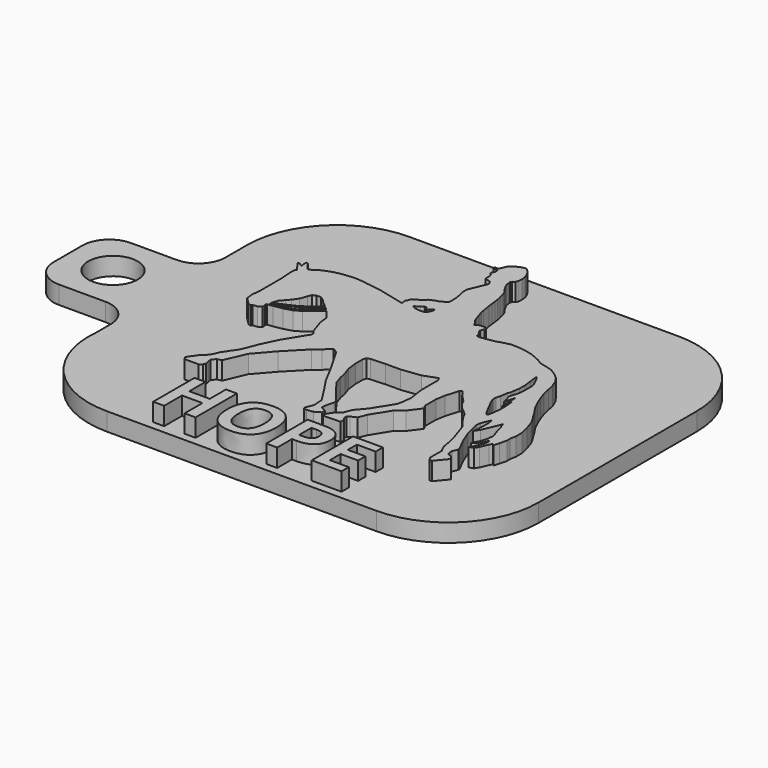
from build123d import *

# Parameters (mm, degrees)
F0_R         = 2.75
F1_DEPTH     = 2
F3_TEXT_SIZE = 8.0529393421
F4_DEPTH     = 2
F5_DEPTH     = 2


# Not quite as in the source:
# - Text() gives the source's letters only with a copy of the font that has no kerning and outlines rounded to 1/6400 em; it was checked with that copy


with BuildPart() as f1:
    # F0 (on Top) → F1 (new body)
    with BuildSketch(Plane.XY):
        with BuildLine():
            ThreePointArc((-13.1507226788, -10), (-10.6170467948, -17.7082039325), (-3.2008483077, -21))
            Line((-3.2008483077, -21), (26.7991516923, -21))
            ThreePointArc((26.7991516923, -21), (33.8702195042, -18.0710678119), (36.7991516923, -11))
            Line((36.7991516923, -11), (36.7991516923, 11))
            ThreePointArc((36.7991516923, 11), (33.8702195042, 18.0710678119), (26.7991516923, 21))
            Line((26.7991516923, 21), (-3.2008483077, 21))
            ThreePointArc((-3.2008483077, 21), (-10.2719161196, 18.0710678119), (-13.2008483077, 11))
            Line((-13.2008483077, 11), (-13.2008483077, 8))
            ThreePointArc((-13.2008483077, 8), (-14.0795279641, 5.8786796564), (-16.2008483077, 5))
            Line((-16.2008483077, 5), (-21.3089559265, 5))
            ThreePointArc((-21.3089559265, 5), (-23.43027627, 4.1213203436), (-24.3089559265, 2))
            Line((-24.3089559265, 2), (-24.3089559265, -2))
            ThreePointArc((-24.3089559265, -2), (-23.43027627, -4.1213203436), (-21.3089559265, -5))
            Line((-21.3089559265, -5), (-16.1507226788, -5))
            ThreePointArc((-16.1507226788, -5), (-14.0294023352, -5.8786796564), (-13.1507226788, -8))
            Line((-13.1507226788, -8), (-13.1507226788, -10))
        make_face()
        with Locations((-19.3089559265, 0)):
            Circle(F0_R, mode=Mode.SUBTRACT)
    extrude(amount=F1_DEPTH)

    # F3 (on face) → F4 (join)
    with BuildSketch(Plane.XY.offset(2)):
        with Locations((0.5135238171, -20.096231252)):
            Text('HOPE', F3_TEXT_SIZE, font='Open Sans', font_style=FontStyle.BOLD, text_align=(TextAlign.LEFT, TextAlign.BOTTOM))
    extrude(amount=F4_DEPTH)

    # F2 (on face) → F5 (join)
    with BuildSketch(Plane.XY.offset(2)):
        Polygon((14.4057357684, -12.9295000806), (16.3045506924, -12.8705985844), (16.2954782047, -12.3983173033), (16.0806663334, -12.0984232053), (16.0806663334, -11.8137812242), (16.300862655, -11.6041181609), (16.9360265136, -11.3009717315), (17.3037418711, -10.3799057515), (18.5667234945, -8.336847648), (19.4170251489, -7.6700611971), (20.3772753385, -6.3978997059), (20.1262235641, -5.9626172297), (20.1262235641, -4.43818653), (20.2957785632, -3.396378751), (20.734641701, -1.9284236478), (20.9365651874, -1.7577570332), (21.4741043746, -2.4432395585), (22.2038775682, -3.195283236), (22.4202004258, -3.6323247982), (22.9209531099, -4.2708963156), (23.7911492586, -4.9933143891), (24.1744478729, -5.7404879736), (25.1152147488, -6.9401758645), (25.5047673759, -8.102159261), (25.8359651324, -9.0900778816), (26.0207999805, -9.8925542569), (26.1829775535, -10.8235611911), (26.3887103647, -11.3350939359), (26.5676892823, -11.6454139352), (26.5676892823, -13.2674037658), (26.7900731415, -13.6529807933), (27.0690526813, -13.6529807933), (28.1546071398, -12.3415887356), (27.8195337628, -11.91429534), (27.6246890426, -11.9076147676), (27.4183303118, -11.7746600881), (27.3406576146, -11.6189256126), (27.289854211, -11.3983582705), (27.289854211, -11.1325758151), (27.5425345508, -10.546027472), (27.5135968314, -10.3799057515), (26.8309513895, -9.0288437401), (26.2567778986, -7.6012224477), (26.0578238236, -6.7374462358), (25.8793570101, -5.9626172297), (25.9441418617, -5.4701659828), (26.3887103647, -4.43818653), (26.4952767074, -5.1568056859), (26.4448728412, -6.6268783994), (26.3512693346, -7.0590674877), (26.7444010824, -6.4693694003), (27.5868289173, -4.4288262725), (27.7840252444, -4.9476545199), (28.0780084431, -5.9626172297), (28.3293427293, -6.6593339926), (28.2371323556, -7.4789840728), (28.001123842, -8.18628259), (27.6055055558, -8.91732222), (28.0312057585, -8.5834981874), (28.3802725508, -8.18628259), (28.5535737633, -7.6066066558), (28.6533644503, -7.610028144), (28.6533644503, -8.18628259), (28.1435307115, -9.3697626144), (27.918882668, -9.6224909648), (28.4013585813, -9.4954507706), (28.6819663905, -9.0415264633), (29.050398618, -8.18628259), (29.2314309627, -7.8517636284), (29.4054470205, -8.0243692113), (29.5858703554, -7.4208704612), (29.7829452902, -6.6268783994), (29.7763942349, -6.1731628859), (29.8888737889, -5.4701659828), (29.8888737889, -4.6576105355), (29.6704190609, -3.7091705624), (29.3347928673, -2.7080425061), (29.0434602648, -2.1314497571), (28.7286803838, -1.6768321487), (28.2960847475, -0.9267824817), (27.8613511473, -0.3198605264), (27.3939305483, 0.6458187127), (27.0699299872, 1.4514116338), (26.8065321311, 2.2446609869), (26.5914796644, 3.17832975), (26.4157085241, 3.9414552589), (26.0975691721, 4.7324749074), (25.7041398436, 5.2817328833), (25.1186332892, 5.7565801296), (24.4813356549, 6.150546018), (23.8515025278, 6.3388423371), (22.9791355302, 6.5553705336), (22.3837151171, 6.9234486801), (21.3705125394, 7.3599282554), (20.5815926346, 7.5557442418), (19.7165142745, 7.6941568404), (18.8413587665, 7.7241629896), (18.1382677906, 7.5622196381), (17.2448255293, 7.3034347474), (16.3118303177, 7.1409108247), (15.8028327753, 7.0781577004), (15.4516413608, 7.117666623), (15.3766200171, 7.376674167), (15.2874930965, 7.5982787718), (15.0793138891, 7.8889131546), (15.0296255656, 8.0652720289), (15.0862894952, 8.2935644314), (15.1866925525, 8.5351212571), (15.1628451422, 8.7285502439), (15.0607703254, 8.8532911029), (14.6830938756, 8.8532911029), (14.3462475389, 8.8090412319), (13.9642081238, 8.6108921573), (13.9168873429, 8.7285502439), (13.7182632894, 9.0058448879), (13.5212177411, 9.257121973), (13.3323129267, 9.7268136943), (13.1886444769, 10.2228220367), (12.9617797656, 10.8995291345), (12.9220215604, 11.222012341), (12.7522886811, 12.1963917492), (12.6947659129, 12.6629652935), (12.6373895197, 13.1283515742), (12.5825373734, 13.5732634076), (12.4628860503, 14.0927399082), (12.3358950912, 14.6440820693), (12.184023687, 15.0216941566), (11.8444845447, 15.4957172366), (11.5512409369, 16.004153411), (11.4555447903, 16.2420916973), (11.4297282051, 16.4514928789), (11.4029068374, 16.6690439634), (11.3867729017, 16.7999081028), (11.4582277826, 16.9657767335), (11.7187928736, 17.1701057165), (11.81913508, 17.4030306642), (11.8690588013, 17.846798328), (11.8006470133, 18.4016939184), (11.6284643142, 18.829807879), (11.3886492327, 19.2456077784), (11.0933948308, 19.5535104722), (10.8797093853, 19.6888073356), (10.5026904296, 19.6423255446), (10.0986134797, 19.4798102654), (9.6864081913, 19.2420683973), (9.4014372543, 19.0186009269), (9.0297050774, 18.1556968618), (8.6688981794, 18.1556968618), (8.575363435, 18.101750138), (8.5913146254, 17.9723682655), (8.8844563685, 17.925465566), (9.1159679477, 17.8994205868), (9.1672958909, 17.7717991173), (9.1672958909, 17.4858884987), (9.0056583988, 17.2244161367), (9.0056583988, 17.1079486746), (9.0216090903, 17.0386973768), (9.2548581452, 16.8271699), (9.2950100008, 16.501493752), (9.2950100008, 16.0436237693), (9.3934232773, 15.9181248609), (9.8117959588, 15.871058067), (9.9814711139, 15.7979633659), (10.1616944747, 15.3498571551), (9.9239231119, 14.7979171072), (9.334008789, 13.428545557), (9.334008789, 12.7822692709), (9.533021627, 11.9182379339), (9.5952630636, 11.4133907482), (9.5952630636, 11.1038507894), (9.5952630636, 10.5683606976), (8.8377370251, 10.1314530193), (8.4686949849, 10.0464513525), (7.862482393, 9.7754532312), (7.773434688, 9.5687462755), (7.1687237712, 9.2199756336), (6.6696759257, 8.9321468007), (6.5858433046, 8.5943948905), (6.4547806883, 8.3823818766), (6.5029077057, 7.992018307), (6.5264196133, 7.8899393401), (6.3388443612, 7.9110414964), (5.2770058221, 8.1745979864), (4.3924666627, 8.3941474071), (3.5704599901, 8.5981757837), (2.6782433787, 8.7409305045), (1.9472041167, 8.8231721893), (1.1549399933, 8.9499345049), (0.4360472958, 8.9999223128), (-0.3550298657, 8.9431121583), (-1.083578395, 8.8532911029), (-1.7623456147, 8.6969502562), (-2.4313051254, 8.4726829082), (-3.0800345292, 8.1745979864), (-3.5510911003, 7.837183732), (-3.8549916855, 7.735301664), (-4.5147598108, 8.5766533857), (-4.6581168893, 8.6652741428), (-4.7388332486, 8.5347035874), (-4.6581168893, 7.8800042569), (-5.1091981368, 8.1588545378), (-5.2491402967, 8.1745979864), (-5.2741511807, 8.0738320349), (-4.9507311765, 7.6613992925), (-4.4976170656, 7.0835775961), (-4.6094932536, 6.9026014455), (-4.6581168893, 6.4703901298), (-4.5513651165, 5.0638681278), (-4.5513651165, 3.0954778194), (-4.5513651165, 1.9436620058), (-4.6581168893, 0.9947546798), (-4.5619914308, 0.2150704386), (-3.7474798462, -0.5943234321), (-3.4712990843, -0.6253936801), (-3.3903366707, -0.4944250957), (-2.8851934087, -0.4321471566), (-2.5077828025, -0.2144733298), (-2.5077828025, -0.0057062971), (-2.5319425578, 0.0991853563), (-2.5757992459, 0.2300039925), (-2.5077828025, 0.3878909582), (-1.9108937122, 0.4614800273), (-0.8987553301, 0.6458187127), (0, 0.9061425298), (0.7114020668, 1.3164479313), (2.3607970983, 2.6098645129), (3.1293474968, 1.629791096), (3.2593631487, 0.5752197428), (3.7923315989, -1.0145538767), (4.0943801749, -1.3997332749), (4.0632066396, -1.6768321487), (2.5680158287, -4.0955226868), (1.6779805301, -5.9481193312), (0.9921386372, -7.6900362037), (0.5374790689, -8.336847648), (-0.0548549726, -9.2235639258), (-0.431542634, -10.097971186), (-1.0948275449, -10.7212318107), (-1.8477179687, -11.7997636751), (-1.6525899991, -12.1380834737), (-0.0900417419, -12.1380834737), (0.2038573346, -11.9076147676), (0.3361684251, -11.6004802633), (0.2267933478, -11.1256189671), (0.1865181403, -10.7989422977), (0.5374790689, -10.3799057515), (1.0402089683, -10.2641116828), (2.0574387163, -7.9028103501), (3.7640798837, -5.9423525818), (5.8369720424, -3.8145952286), (6.5262070857, -3.2741134055), (7.2511202059, -2.5279033566), (7.8156586153, -2.8768908061), (9.2243542895, -5.3193373606), (10.4674790055, -7.6557914726), (11.4393364638, -9.1057261452), (12.4628860503, -10.7212318107), (12.542760931, -11.8435025215), (12.1880317868, -12.704298012), (12.2453598306, -12.8752999008), (12.5538124515, -12.9654358891), (13.2664684206, -12.8775741905), (13.9168873429, -12.5024411827), (13.9168873429, -12.0695345104), (13.5212177411, -11.9076147676), (13.3323129267, -11.7698712274), (13.3323129267, -11.4510944113), (13.5909453758, -10.4090942619), (13.5491946712, -10.0704496726), (13.0443628877, -9.4802035019), (12.1477702633, -8.336847648), (11.3876733474, -7.2756931705), (11.0933948308, -6.3978997059), (10.8797093853, -5.4701659828), (10.6073017845, -4.6576105355), (10.4674790055, -3.5234924871), (10.4674790055, -2.5159725919), (10.5888666585, -2.1214617882), (10.9651694074, -2.0304208156), (12.5497952104, -1.9438075833), (14.2243178561, -1.9438075833), (16.3319073617, -1.6839677701), (17.8187675774, -1.1354173766), (18.035300076, -1.4241281897), (18.035300076, -2.4634872098), (18.035300076, -3.8781699259), (18.2807035744, -5.523821339), (18.1507840753, -6.6786645912), (18.035300076, -7.1839080192), (16.6555959731, -9.395503439), (15.7172307372, -10.4874065146), (15.3705142438, -11.3918855786), (14.8881245404, -11.7235276848), (14.4660342485, -12.3415887356), (14.2097650096, -12.756141834), align=None)
        Polygon((0.7803506547, 2.1377503983), (1.9207079895, 3.031991655), (2.1353650372, 2.8217774816), (0.7837259327, 1.6832037363), (-0.0899588704, 1.1401023949), (-1.0226764716, 0.8173899841), (-2.3492628576, 0.6119563146), (-2.3961719126, 0.671775837), (-1.1930471958, 1.0943717908), (0, 1.6577552306), align=None, mode=Mode.SUBTRACT)
        Polygon((1.1432619067, 3.6654123105), (1.7351189163, 3.2034749165), (0.6813245127, 2.3806493264), (-0.1848077227, 1.8176630838), (-1.2241665972, 1.32685469), (-2.3790099658, 0.8360464708), (-2.2923967335, 1.1103216093), (-2.1480412688, 1.5145167708), (-1.7294107238, 1.9908896647), (-1.3685221784, 2.3950848263), (-0.9643269004, 2.9725064524), (-0.6756162038, 3.7664610427), (-0.5312606809, 4.1562207043), (-0.170372412, 4.3583181687), (0.3348715545, 4.3583181687), (0.7535022451, 4.0696072392), align=None, mode=Mode.SUBTRACT)
        Polygon((24.4098696858, 3.3528357744), (24.2892727256, 4.340225365), (24.5670415461, 4.0296907537), (25.0918439426, 2.8699815739), (25.0918439426, 1.5219721154), (25.0096600503, 0.8949868497), (24.7353836894, 0), (25.0240955502, -1.1115532834), (25.3621570743, 0.1443387882), (25.3621570743, -1.387183881), (25.4214515174, -1.872658107), (25.5703758788, -0.7365062685), (25.6655771071, -1.5159678878), (25.6655771071, -2.4406380654), (25.5089618328, -3.6354642858), (25.3702756017, -3.9128381759), (25.2798274159, -3.8676143158), (25.0461716205, -3.5058225039), (24.7672889382, -2.993284259), (24.4733337313, -2.4053726811), (24.1643041372, -1.8099236768), (24.0099542238, -1.421617407), (23.9832717925, -1.203154563), (23.9832717925, -0.8854765911), (24.134779349, -0.4260654678), (24.2441445589, 0.4082875093), (24.3614409119, 0.6477677962), (24.4098696858, 0.9801078122), (24.5159745731, 1.7021608073), (24.5159745731, 2.4841002683), align=None, mode=Mode.SUBTRACT)
        Polygon((8.1236521938, 7.7901966401), (7.6727932319, 7.9844230786), (7.6877626829, 8.1009697261), (7.9073859379, 8.1745979864), (8.2006277516, 8.3607491106), (8.4058959037, 8.5220318288), (8.5231922567, 8.6002293974), (8.6893625557, 8.5904542357), (8.7382365018, 8.4927072749), (8.7871095166, 8.2825515419), (8.9679416269, 8.2972133532), (9.3393492523, 8.6468040845), (9.4908885658, 8.70775152), (9.533021627, 8.6002293974), (9.4322403893, 8.2287909463), (9.2562958598, 7.8573515639), (8.9826034382, 7.7693792991), (8.5329674184, 7.7547174878), align=None, mode=Mode.SUBTRACT)
    extrude(amount=F5_DEPTH)


solid = f1.part
